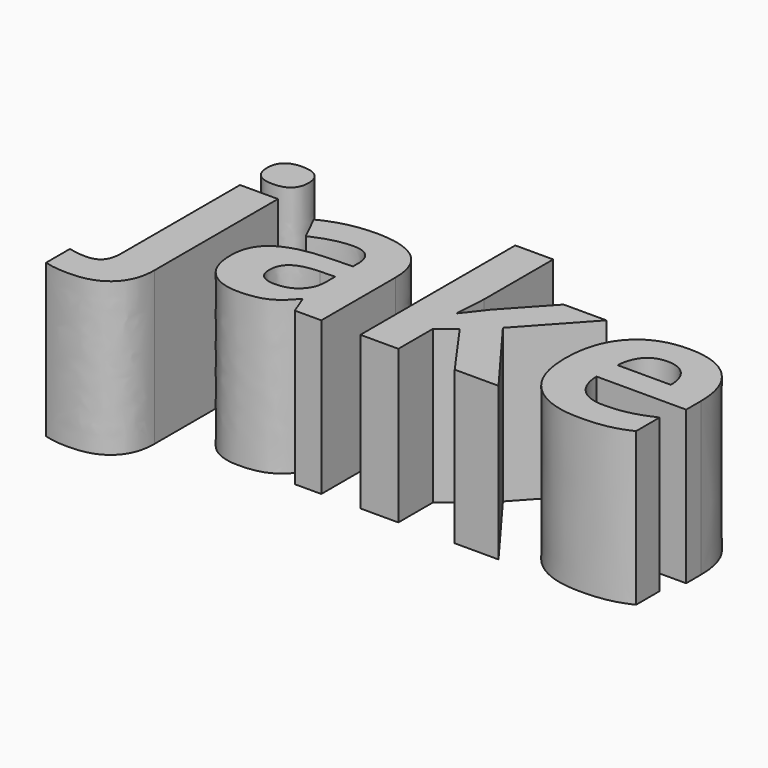
from build123d import *

# Parameters (mm, degrees)
F0_TEXT_SIZE = 42.3333342446
F1_DEPTH     = 25.4


# Not quite as in the source:
# - Text() gives the source's letters only with a copy of the font that has no kerning and outlines rounded to 1/6400 em; it was checked with that copy


with BuildPart() as f1:
    # F0 (on Top) → F1 (new body)
    with BuildSketch(Plane.XY):
        with Locations((-26.5175998211, -4.4196001254)):
            Text('jake', F0_TEXT_SIZE, font='Open Sans', font_style=FontStyle.BOLD, text_align=(TextAlign.LEFT, TextAlign.BOTTOM))
    extrude(amount=F1_DEPTH)


solid = f1.part
